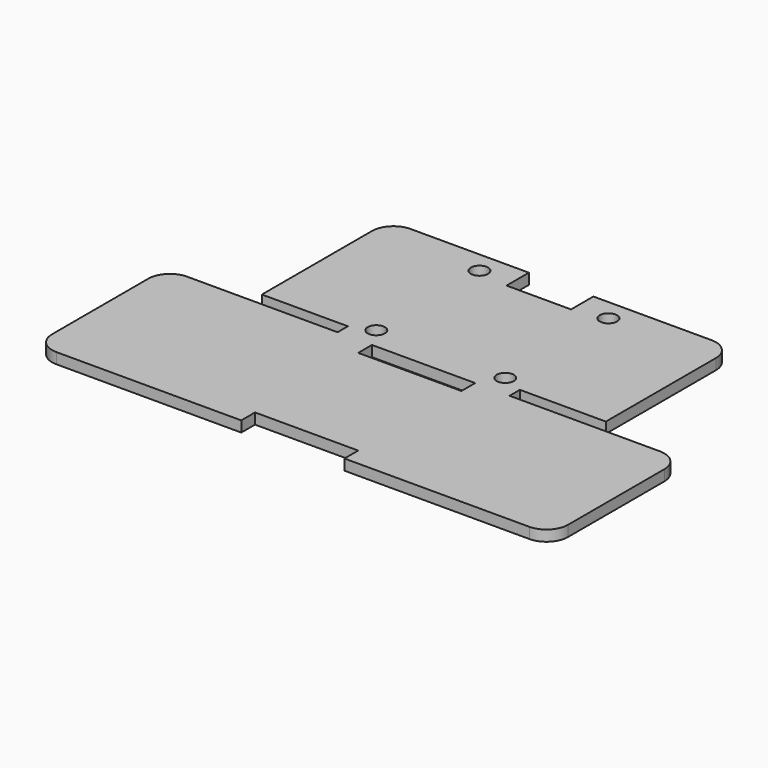
from build123d import *

# Parameters (mm, degrees)
F0_W     = 24
F0_H     = 4
F0_R     = 2
F1_DEPTH = 2.5
F2_W     = 20
F2_H     = 3
F3_DEPTH = 25
F4_SIZE  = 2.49999


# Not quite as in the source:
# - a fillet or chamfer is up to 0.001 mm smaller than in the source, because OpenCascade refuses the exact size


with BuildPart() as f1:
    # F0 (on Top) → F1 (new body)
    with BuildSketch(Plane.XY):
        with BuildLine():
            Line((-36.8828806926, 6.1976464093), (-51.8828806926, 6.1976464093))
            ThreePointArc((-51.8828806926, 6.1976464093), (-55.4184145986, 4.7331803152), (-56.8828806926, 1.1976464093))
            Line((-56.8828806926, 1.1976464093), (-56.8828806926, -26.8023535907))
            ThreePointArc((-56.8828806926, -26.8023535907), (-55.4184145986, -30.3378874967), (-51.8828806926, -31.8023535907))
            Line((-51.8828806926, -31.8023535907), (-8.8828806926, -31.8023535907))
            Line((-8.8828806926, -31.8023535907), (-8.8828806926, -27.8023535907))
            Line((-8.8828806926, -27.8023535907), (15.1171193074, -27.8023535907))
            Line((15.1171193074, -27.8023535907), (15.1171193074, -31.8023535907))
            Line((15.1171193074, -31.8023535907), (58.1171193074, -31.8023535907))
            ThreePointArc((58.1171193074, -31.8023535907), (61.6526532133, -30.3378874967), (63.1171193074, -26.8023535907))
            Line((63.1171193074, -26.8023535907), (63.1171193074, 1.1976464093))
            ThreePointArc((63.1171193074, 1.1976464093), (61.6526532133, 4.7331803152), (58.1171193074, 6.1976464093))
            Line((58.1171193074, 6.1976464093), (43.1171193074, 6.1976464093))
            Line((43.1171193074, 6.1976464093), (23.1171193074, 6.1976464093))
            Line((23.1171193074, 6.1976464093), (23.1171193074, 41.1976464093))
            ThreePointArc((23.1171193074, 41.1976464093), (21.6526532133, 44.7331803152), (18.1171193074, 46.1976464093))
            Line((18.1171193074, 46.1976464093), (10.6171193074, 46.1976464093))
            Line((10.6171193074, 46.1976464093), (10.6171193074, 42.1976464093))
            Line((10.6171193074, 42.1976464093), (-4.3828806926, 42.1976464093))
            Line((-4.3828806926, 42.1976464093), (-4.3828806926, 46.1976464093))
            Line((-4.3828806926, 46.1976464093), (-11.8828806926, 46.1976464093))
            ThreePointArc((-11.8828806926, 46.1976464093), (-15.4184145986, 44.7331803152), (-16.8828806926, 41.1976464093))
            Line((-16.8828806926, 41.1976464093), (-16.8828806926, 6.1976464093))
            Line((-16.8828806926, 6.1976464093), (-36.8828806926, 6.1976464093))
        make_face()
        with Locations((3.1171193074, 4.1976464093)):
            Rectangle(F0_W, F0_H, mode=Mode.SUBTRACT)
        with Locations((-11.8828806926, 11.1976464093)):
            Circle(F0_R, mode=Mode.SUBTRACT)
        with Locations((-11.8828806926, 41.1976464093)):
            Circle(F0_R, mode=Mode.SUBTRACT)
        with Locations((18.1171193074, 11.1976464093)):
            Circle(F0_R, mode=Mode.SUBTRACT)
        with Locations((18.1171193074, 41.1976464093)):
            Circle(F0_R, mode=Mode.SUBTRACT)
        with BuildLine():
            Line((-36.8828806926, 41.1976464093), (-36.8828806926, 6.1976464093))
            Line((-36.8828806926, 6.1976464093), (-16.8828806926, 6.1976464093))
            Line((-16.8828806926, 6.1976464093), (-16.8828806926, 41.1976464093))
            ThreePointArc((-16.8828806926, 41.1976464093), (-15.4184145986, 44.7331803152), (-11.8828806926, 46.1976464093))
            Line((-11.8828806926, 46.1976464093), (-16.8828806926, 46.1976464093))
            Line((-16.8828806926, 46.1976464093), (-31.8828806926, 46.1976464093))
            ThreePointArc((-31.8828806926, 46.1976464093), (-35.4184145986, 44.7331803152), (-36.8828806926, 41.1976464093))
        make_face()
        with BuildLine():
            Line((23.1171193074, 46.1976464093), (18.1171193074, 46.1976464093))
            ThreePointArc((18.1171193074, 46.1976464093), (21.6526532133, 44.7331803152), (23.1171193074, 41.1976464093))
            Line((23.1171193074, 41.1976464093), (23.1171193074, 6.1976464093))
            Line((23.1171193074, 6.1976464093), (43.1171193074, 6.1976464093))
            Line((43.1171193074, 6.1976464093), (43.1171193074, 41.1976464093))
            ThreePointArc((43.1171193074, 41.1976464093), (41.6526532133, 44.7331803152), (38.1171193074, 46.1976464093))
            Line((38.1171193074, 46.1976464093), (23.1171193074, 46.1976464093))
        make_face()
    extrude(amount=F1_DEPTH)

    # F2 (on face) → F3 (cut)
    with BuildSketch(Plane.XY.offset(2.5)):
        with Locations((-26.8828806926, 7.6976464093)):
            Rectangle(F2_W, F2_H)
        with Locations((33.1171193074, 7.6976464093)):
            Rectangle(F2_W, F2_H)
    extrude(amount=-F3_DEPTH, mode=Mode.SUBTRACT)

    # F4 (size 2.5 in the source; OpenCascade refuses exactly that, so slightly less here)
    f4_edges = [f1.edges().sort_by_distance(p)[0] for p in [
        (3.117119, 42.197646, 2.5),
    ]]
    chamfer(f4_edges, length=F4_SIZE)


solid = f1.part
